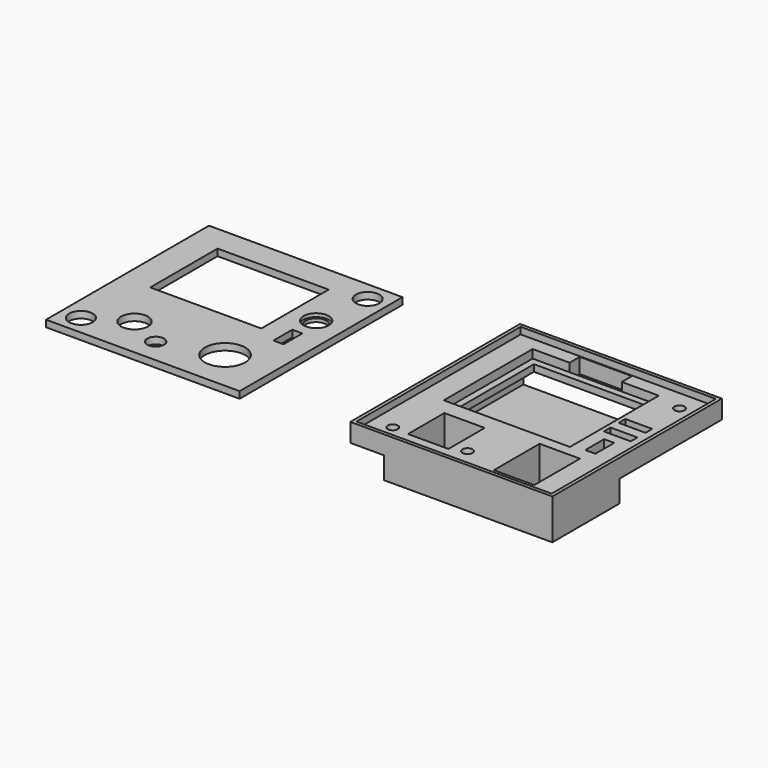
from build123d import *

# Parameters (mm, degrees)
F1_W      = 60
F1_H      = 63
F1_R      = 1.5
F1_W_2    = 3
F1_H_2    = 7
F1_W_3    = 37.5
F1_H_3    = 33
F1_W_4    = 12
F1_H_4    = 8
F1_W_5    = 8
F1_H_5    = 3
F2_DEPTH  = 3.5
F4_W      = 37.5
F4_H      = 33
F4_W_2    = 33.5
F4_H_2    = 29
F5_DEPTH  = 1
F3_W      = 15.5
F3_H      = 3.75
F6_DEPTH  = 2.5
F0_W      = 57.5
F0_H      = 60.5
F0_R      = 3.5
F0_R_2    = 2.5
F0_R_3    = 4
F0_R_4    = 6
F0_W_2    = 3
F0_H_2    = 7
F0_W_3    = 33
F0_H_3    = 25
F0_R_5    = 3.1
F8_DEPTH  = 2
F10_W     = 46
F10_H     = 38
F11_DEPTH = 11
F12_W     = 44
F12_H     = 9
F13_DEPTH = 37
F14_W     = 1
F14_H     = 5
F15_DEPTH = 20
F16_W     = 33.5
F16_H     = 29
F16_W_2   = 15.5
F16_H_2   = 3.75
F17_DEPTH = 4
F18_W     = 60
F18_H     = 63
F18_W_2   = 58
F18_H_2   = 61
F19_DEPTH = 2
F20_W     = 50
F20_H     = 25
F20_W_2   = 12
F20_H_2   = 2.75
F20_H_3   = 4.5
F20_R     = 1.5
F21_DEPTH = 6.5
F22_W     = 12
F22_H     = 13.5
F22_H_2   = 17
F23_DEPTH = 9
F26_R     = 3.75
F27_DEPTH = 1


# Not quite as in the source:
# - a feature names something its author has since deleted; it is built from what else it names


with BuildPart() as f2:
    # F1 (on Top) → F2 (new body)
    with BuildSketch(Plane.XY):
        with Locations((92.6610440163, 0)):
            Rectangle(F1_W, F1_H)
        with Locations((69.6610440163, -24.5)):
            Circle(F1_R, mode=Mode.SUBTRACT)
        Polygon((86.5110440163, -22.15), (86.5110440163, -24.9), (74.5110440163, -24.9), (74.5110440163, -22.15), (74.5110440163, -14.15), (74.5110440163, -11.4), (86.5110440163, -11.4), (86.5110440163, -14.15), align=None, mode=Mode.SUBTRACT)
        with Locations((90.6610440163, -23)):
            Circle(F1_R, mode=Mode.SUBTRACT)
        Polygon((113.4110440163, -22.15), (113.4110440163, -26.65), (101.4110440163, -26.65), (101.4110440163, -22.15), (101.4110440163, -14.15), (101.4110440163, -9.65), (113.4110440163, -9.65), (113.4110440163, -14.15), align=None, mode=Mode.SUBTRACT)
        with Locations((113.1610440163, -2)):
            Rectangle(F1_W_2, F1_H_2, mode=Mode.SUBTRACT)
        with Locations((89.1610440163, 10)):
            Rectangle(F1_W_3, F1_H_3, mode=Mode.SUBTRACT)
        Polygon((117.1610440163, 7), (117.1610440163, 4.5), (109.1610440163, 4.5), (109.1610440163, 7), (109.1610440163, 10), (109.1610440163, 12.5), (117.1610440163, 12.5), (117.1610440163, 10), align=None, mode=Mode.SUBTRACT)
        with Locations((115.6610440163, 24.5)):
            Circle(F1_R, mode=Mode.SUBTRACT)
        with Locations((80.5110440163, -18.15)):
            Rectangle(F1_W_4, F1_H_4)
        with Locations((107.4110440163, -18.15)):
            Rectangle(F1_W_4, F1_H_4)
        with Locations((113.1610440163, 8.5)):
            Rectangle(F1_W_5, F1_H_5)
    extrude(amount=F2_DEPTH)

    # F4 (on face) → F5 (join)
    with BuildSketch(Plane(origin=(0, 0, 0), x_dir=(1, 0, 0), z_dir=(0, 0, -1))):
        with Locations((89.1610440163, -10)):
            Rectangle(F4_W, F4_H)
        with Locations((89.1610440163, -10)):
            Rectangle(F4_W_2, F4_H_2, mode=Mode.SUBTRACT)
    extrude(amount=-F5_DEPTH)

    # F3 (on face) → F6 (cut)
    with BuildSketch(Plane.XY.offset(3.5)):
        with Locations((89.1610440163, 28.375)):
            Rectangle(F3_W, F3_H)
    extrude(amount=-F6_DEPTH, mode=Mode.SUBTRACT)

    # F10 (on face) → F11 (join)
    with BuildSketch(Plane(origin=(0, 0, 0), x_dir=(1, 0, 0), z_dir=(0, 0, -1))):
        with Locations((85.6610440163, -12.5)):
            Rectangle(F10_W, F10_H)
    extrude(amount=F11_DEPTH)

    # F12 (on face) → F13 (cut)
    with BuildSketch(Plane(origin=(0, 31.5, 0), x_dir=(-1, 0, 0), z_dir=(0, 1, 0))):
        with Locations((-85.6610440163, -5.5)):
            Rectangle(F12_W, F12_H)
    extrude(amount=-F13_DEPTH, mode=Mode.SUBTRACT)

    # F14 (on face) → F15 (cut)
    with BuildSketch(Plane(origin=(0, 31.5, 0), x_dir=(-1, 0, 0), z_dir=(0, 1, 0))):
        with Locations((-108.1610440163, -6.5)):
            Rectangle(F14_W, F14_H)
    extrude(amount=-F15_DEPTH, mode=Mode.SUBTRACT)

    # F16 (on face) → F17 (cut)
    with BuildSketch(Plane.XY.offset(1)):
        with Locations((89.1610440163, 10)):
            Rectangle(F16_W, F16_H)
        with Locations((89.1610440163, 28.375)):
            Rectangle(F16_W_2, F16_H_2)
    extrude(amount=-F17_DEPTH, mode=Mode.SUBTRACT)

    # F18 (on face) → F19 (join)
    with BuildSketch(Plane.XY.offset(3.5)):
        with Locations((92.6610440163, 0)):
            Rectangle(F18_W, F18_H)
        with Locations((92.6610440163, 0)):
            Rectangle(F18_W_2, F18_H_2, mode=Mode.SUBTRACT)
    extrude(amount=F19_DEPTH)

    # F20 (on face) → F21 (join)
    with BuildSketch(Plane(origin=(0, 0, 0), x_dir=(1, 0, 0), z_dir=(0, 0, -1))):
        with Locations((97.6610440163, 19)):
            Rectangle(F20_W, F20_H)
        with Locations((80.5110440163, 12.775)):
            Rectangle(F20_W_2, F20_H_2, mode=Mode.SUBTRACT)
        with Locations((107.4110440163, 11.9)):
            Rectangle(F20_W_2, F20_H_3, mode=Mode.SUBTRACT)
        with Locations((80.5110440163, 23.525)):
            Rectangle(F20_W_2, F20_H_2, mode=Mode.SUBTRACT)
        with Locations((90.6610440163, 23)):
            Circle(F20_R, mode=Mode.SUBTRACT)
        with Locations((107.4110440163, 24.4)):
            Rectangle(F20_W_2, F20_H_3, mode=Mode.SUBTRACT)
    extrude(amount=F21_DEPTH)

    # F22 (on face) → F23 (cut)
    with BuildSketch(Plane.XY.offset(3.5)):
        with Locations((80.5110440163, -18.15)):
            Rectangle(F22_W, F22_H)
        with Locations((107.4110440163, -18.15)):
            Rectangle(F22_W, F22_H_2)
    extrude(amount=-F23_DEPTH, mode=Mode.SUBTRACT)


with BuildPart() as f8:
    # F0 (on Top) → F8 (new body)
    with BuildSketch(Plane.XY):
        Rectangle(F0_W, F0_H)
        with Locations((-23, -24.5)):
            Circle(F0_R, mode=Mode.SUBTRACT)
        with Locations((-2, -23)):
            Circle(F0_R_2, mode=Mode.SUBTRACT)
        with Locations((-12.15, -18.15)):
            Circle(F0_R_3, mode=Mode.SUBTRACT)
        with Locations((14.75, -18.15)):
            Circle(F0_R_4, mode=Mode.SUBTRACT)
        with Locations((20.5, -2)):
            Rectangle(F0_W_2, F0_H_2, mode=Mode.SUBTRACT)
        with Locations((-3.5, 10)):
            Rectangle(F0_W_3, F0_H_3, mode=Mode.SUBTRACT)
        with Locations((20.5, 8.5)):
            Circle(F0_R_5, mode=Mode.SUBTRACT)
        with Locations((23, 24.5)):
            Circle(F0_R, mode=Mode.SUBTRACT)
    extrude(amount=F8_DEPTH)

    # F26 (on face) → F27 (cut)
    with BuildSketch(Plane.XY.offset(2)):
        with Locations((20.5, 8.5)):
            Circle(F26_R)
    extrude(amount=-F27_DEPTH, mode=Mode.SUBTRACT)


solid = Compound([f2.part, f8.part])
